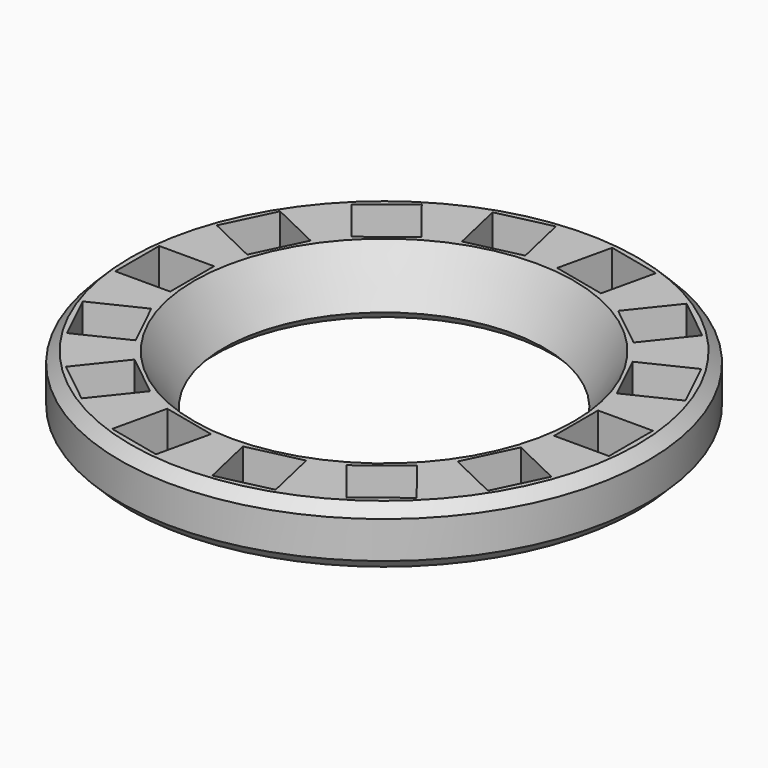
from build123d import *

# Parameters (mm, degrees)
F0_R     = 25
F0_W     = 5.2
F0_H     = 5.2
F0_R_2   = 15
F1_DEPTH = 5
F2_DEPTH = 0.5
F3_SIZE2 = 2.99999
F3_SIZE  = 4.99999


# Not quite as in the source:
# - a fillet or chamfer that OpenCascade refuses, or shapes differently, is made with other operations: its cross-section is extruded or revolved along the edge and cut away or added
# - a fillet or chamfer is up to 0.001 mm smaller than in the source, because OpenCascade refuses the exact size


with BuildPart() as f1:
    # F0 (on Top) → F1 (new body)
    with BuildSketch(Plane.XY):
        Circle(F0_R)
        Polygon((-12.7365232116, -19.9005898526), (-16.8020469205, -16.6584428829), (-13.5598999508, -12.5929191741), (-9.494376242, -15.8350661437), align=None, mode=Mode.SUBTRACT)
        Polygon((-2.8406685631, -23.4559822245), (-7.9102937065, -22.2988733679), (-6.7531848499, -17.2292482245), (-1.6835597066, -18.3863570811), align=None, mode=Mode.SUBTRACT)
        Polygon((-20.1097532349, -12.4036415956), (-22.3659486783, -7.7186034825), (-17.6809105652, -5.4624080391), (-15.4247151218, -10.1474461522), align=None, mode=Mode.SUBTRACT)
        Polygon((7.6178153328, -22.3656296481), (2.5481901895, -23.5227385047), (1.3910813329, -18.4531133613), (6.4607064762, -17.2960045047), align=None, mode=Mode.SUBTRACT)
        Polygon((16.5674974757, -16.8454898234), (12.5019737669, -20.0876367931), (9.2598267972, -16.0221130843), (13.3253505061, -12.7799661146), align=None, mode=Mode.SUBTRACT)
        Polygon((22.2357835565, -7.9888941429), (19.9795881131, -12.673932256), (15.29455, -10.4177368126), (17.5507454435, -5.7326986995), align=None, mode=Mode.SUBTRACT)
        with Locations((20.9, -0.15)):
            Rectangle(F0_W, F0_H, mode=Mode.SUBTRACT)
        with Locations((-20.9, 0.15)):
            Rectangle(F0_W, F0_H, mode=Mode.SUBTRACT)
        Polygon((-22.2357835565, 7.9888941429), (-19.9795881131, 12.673932256), (-15.29455, 10.4177368126), (-17.5507454435, 5.7326986995), align=None, mode=Mode.SUBTRACT)
        Polygon((-16.5674974757, 16.8454898234), (-12.5019737669, 20.0876367931), (-9.2598267972, 16.0221130843), (-13.3253505061, 12.7799661146), align=None, mode=Mode.SUBTRACT)
        Polygon((-7.6178153328, 22.3656296481), (-2.5481901895, 23.5227385047), (-1.3910813329, 18.4531133613), (-6.4607064762, 17.2960045047), align=None, mode=Mode.SUBTRACT)
        Circle(F0_R_2, mode=Mode.SUBTRACT)
        Polygon((20.1097532349, 12.4036415956), (22.3659486783, 7.7186034825), (17.6809105652, 5.4624080391), (15.4247151218, 10.1474461522), align=None, mode=Mode.SUBTRACT)
        Polygon((2.8406685631, 23.4559822245), (7.9102937065, 22.2988733679), (6.7531848499, 17.2292482245), (1.6835597066, 18.3863570811), align=None, mode=Mode.SUBTRACT)
        Polygon((12.7365232116, 19.9005898526), (16.8020469205, 16.6584428829), (13.5598999508, 12.5929191741), (9.494376242, 15.8350661437), align=None, mode=Mode.SUBTRACT)
    extrude(amount=F1_DEPTH)

    # F0 (on Top) → F2 (join)
    with BuildSketch(Plane.XY):
        Circle(F0_R)
        Polygon((-12.7365232116, -19.9005898526), (-16.8020469205, -16.6584428829), (-13.5598999508, -12.5929191741), (-9.494376242, -15.8350661437), align=None, mode=Mode.SUBTRACT)
        Polygon((-2.8406685631, -23.4559822245), (-7.9102937065, -22.2988733679), (-6.7531848499, -17.2292482245), (-1.6835597066, -18.3863570811), align=None, mode=Mode.SUBTRACT)
        Polygon((-20.1097532349, -12.4036415956), (-22.3659486783, -7.7186034825), (-17.6809105652, -5.4624080391), (-15.4247151218, -10.1474461522), align=None, mode=Mode.SUBTRACT)
        Polygon((7.6178153328, -22.3656296481), (2.5481901895, -23.5227385047), (1.3910813329, -18.4531133613), (6.4607064762, -17.2960045047), align=None, mode=Mode.SUBTRACT)
        Polygon((16.5674974757, -16.8454898234), (12.5019737669, -20.0876367931), (9.2598267972, -16.0221130843), (13.3253505061, -12.7799661146), align=None, mode=Mode.SUBTRACT)
        Polygon((22.2357835565, -7.9888941429), (19.9795881131, -12.673932256), (15.29455, -10.4177368126), (17.5507454435, -5.7326986995), align=None, mode=Mode.SUBTRACT)
        with Locations((20.9, -0.15)):
            Rectangle(F0_W, F0_H, mode=Mode.SUBTRACT)
        with Locations((-20.9, 0.15)):
            Rectangle(F0_W, F0_H, mode=Mode.SUBTRACT)
        Polygon((-22.2357835565, 7.9888941429), (-19.9795881131, 12.673932256), (-15.29455, 10.4177368126), (-17.5507454435, 5.7326986995), align=None, mode=Mode.SUBTRACT)
        Polygon((-16.5674974757, 16.8454898234), (-12.5019737669, 20.0876367931), (-9.2598267972, 16.0221130843), (-13.3253505061, 12.7799661146), align=None, mode=Mode.SUBTRACT)
        Polygon((-7.6178153328, 22.3656296481), (-2.5481901895, 23.5227385047), (-1.3910813329, 18.4531133613), (-6.4607064762, 17.2960045047), align=None, mode=Mode.SUBTRACT)
        Circle(F0_R_2, mode=Mode.SUBTRACT)
        Polygon((20.1097532349, 12.4036415956), (22.3659486783, 7.7186034825), (17.6809105652, 5.4624080391), (15.4247151218, 10.1474461522), align=None, mode=Mode.SUBTRACT)
        Polygon((2.8406685631, 23.4559822245), (7.9102937065, 22.2988733679), (6.7531848499, 17.2292482245), (1.6835597066, 18.3863570811), align=None, mode=Mode.SUBTRACT)
        Polygon((12.7365232116, 19.9005898526), (16.8020469205, 16.6584428829), (13.5598999508, 12.5929191741), (9.494376242, 15.8350661437), align=None, mode=Mode.SUBTRACT)
        Polygon((-15.29455, 10.4177368126), (-19.9795881131, 12.673932256), (-22.2357835565, 7.9888941429), (-17.5507454435, 5.7326986995), align=None)
        Polygon((-9.2598267972, 16.0221130843), (-12.5019737669, 20.0876367931), (-16.5674974757, 16.8454898234), (-13.3253505061, 12.7799661146), align=None)
        Polygon((-1.3910813329, 18.4531133613), (-2.5481901895, 23.5227385047), (-7.6178153328, 22.3656296481), (-6.4607064762, 17.2960045047), align=None)
        Polygon((6.7531848499, 17.2292482245), (7.9102937065, 22.2988733679), (2.8406685631, 23.4559822245), (1.6835597066, 18.3863570811), align=None)
        Polygon((13.5598999508, 12.5929191741), (16.8020469205, 16.6584428829), (12.7365232116, 19.9005898526), (9.494376242, 15.8350661437), align=None)
        Polygon((17.6809105652, 5.4624080391), (22.3659486783, 7.7186034825), (20.1097532349, 12.4036415956), (15.4247151218, 10.1474461522), align=None)
        with Locations((20.9, -0.15)):
            Rectangle(F0_W, F0_H)
        Polygon((15.29455, -10.4177368126), (19.9795881131, -12.673932256), (22.2357835565, -7.9888941429), (17.5507454435, -5.7326986995), align=None)
        Polygon((9.2598267972, -16.0221130843), (12.5019737669, -20.0876367931), (16.5674974757, -16.8454898234), (13.3253505061, -12.7799661146), align=None)
        with Locations((-20.9, 0.15)):
            Rectangle(F0_W, F0_H)
        Polygon((-13.5598999508, -12.5929191741), (-16.8020469205, -16.6584428829), (-12.7365232116, -19.9005898526), (-9.494376242, -15.8350661437), align=None)
        Polygon((-17.6809105652, -5.4624080391), (-22.3659486783, -7.7186034825), (-20.1097532349, -12.4036415956), (-15.4247151218, -10.1474461522), align=None)
        Polygon((-6.7531848499, -17.2292482245), (-7.9102937065, -22.2988733679), (-2.8406685631, -23.4559822245), (-1.6835597066, -18.3863570811), align=None)
        Polygon((1.3910813329, -18.4531133613), (2.5481901895, -23.5227385047), (7.6178153328, -22.3656296481), (6.4607064762, -17.2960045047), align=None)
    extrude(amount=-F2_DEPTH)

    # F3 (size 5 and 3 in the source; OpenCascade refuses exactly that, so slightly less here)
    f3_edges = [f1.edges().sort_by_distance(p)[0] for p in [
        (-15, 0, 5),
    ]]
    f3_side = f1.faces().sort_by_distance((-15, 0, 2.5))[0]
    chamfer(f3_edges, length=F3_SIZE, length2=F3_SIZE2, reference=f3_side)

    # F4: chamfer of 1 on 3 edges, made by hand

    # F4_s1 → F4_t2 (revolve, cut)
    with BuildSketch(Plane.XZ):
        Polygon((24, 5), (25, 4), (25, 5), align=None)
    revolve(axis=Axis((0, 0, 5), (0, 0, 1)), mode=Mode.SUBTRACT)

    # F4_s3 → F4_t4 (revolve, cut)
    with BuildSketch(Plane.XZ):
        Polygon((25, 0.5), (24, -0.5), (25, -0.5), align=None)
    revolve(axis=Axis((0, 0, -0.5), (0, 0, 1)), mode=Mode.SUBTRACT)

    # F4_s5 → F4_t6 (revolve, cut)
    with BuildSketch(Plane.XZ):
        Polygon((15, 0.5), (16, -0.5), (15, -0.5), align=None)
    revolve(axis=Axis((0, 0, -0.5), (0, 0, 1)), mode=Mode.SUBTRACT)


solid = f1.part
